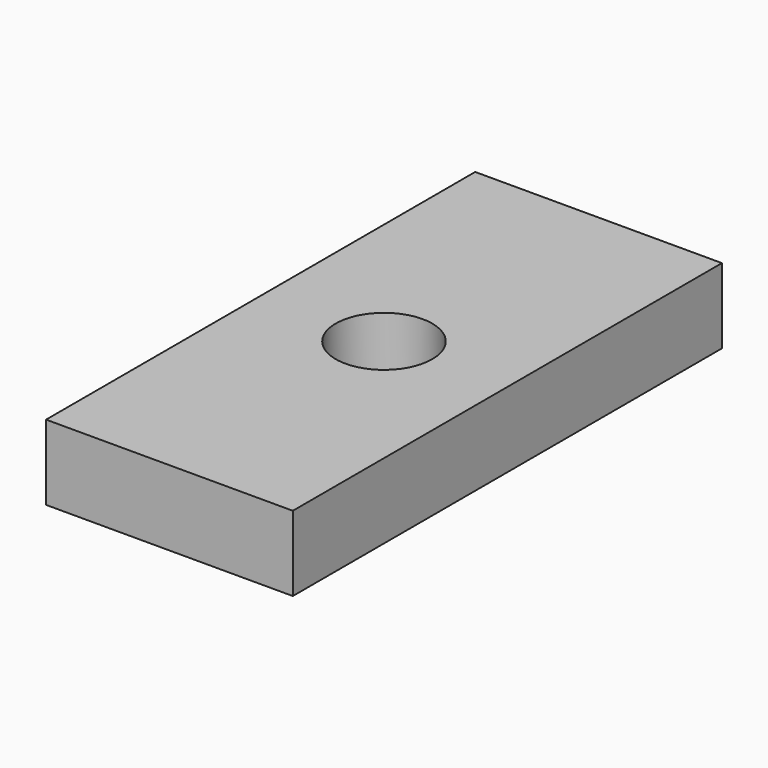
from build123d import *

# Parameters (mm, degrees)
F0_W     = 23
F0_H     = 50
F1_DEPTH = 15
F4_R     = 4.5
F5_DEPTH = 16
F6_W     = 23
F6_H     = 50
F7_DEPTH = 8


# Not quite as in the source:
# - a feature of the source that left no trace in its solid (it failed there, or was rolled back) is left out


with BuildPart() as f1:
    # F0 (on Top) → F1 (new body)
    with BuildSketch(Plane.XY):
        Rectangle(F0_W, F0_H)
    extrude(amount=-F1_DEPTH)

    # F4 (on face) → F5 (cut)
    with BuildSketch(Plane.XY):
        Circle(F4_R)
    extrude(amount=-F5_DEPTH, mode=Mode.SUBTRACT)

    # F6 (on face) → F7 (cut)
    with BuildSketch(Plane.XY):
        Rectangle(F6_W, F6_H)
    extrude(amount=-F7_DEPTH, mode=Mode.SUBTRACT)


solid = f1.part
